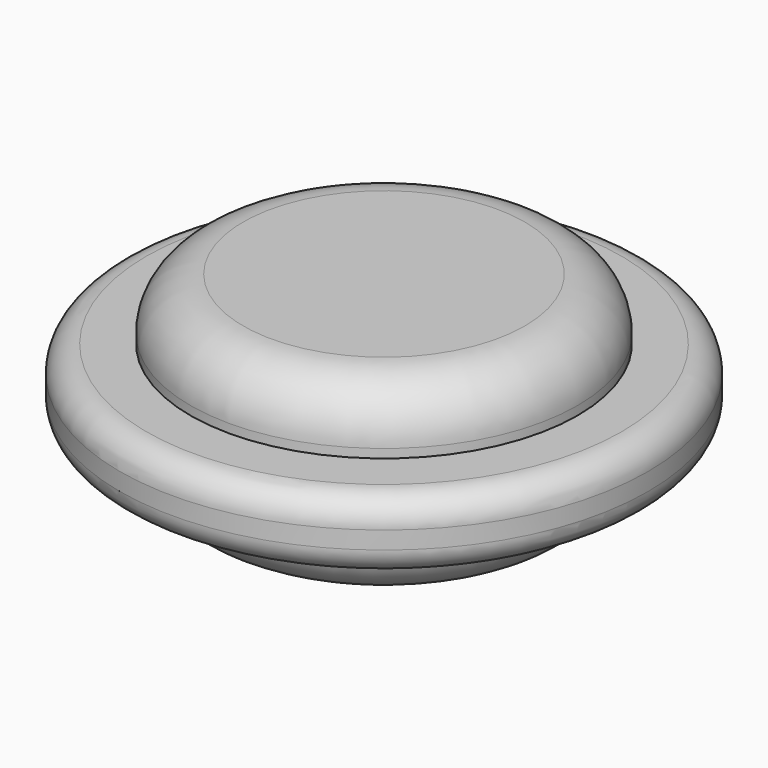
from build123d import *

# Parameters (mm, degrees)
F2_R     = 15
F2_R_2   = 11
F3_DEPTH = 2
F4_R     = 11
F5_DEPTH = 5.5
F6_R     = 3
F7_R     = 1.5
F8_R     = 15
F8_R_2   = 10.75
F9_DEPTH = 2


with BuildPart() as f3:
    # F2 (on Top) → F3 (new body, symmetric)
    with BuildSketch(Plane.XY):
        Circle(F2_R)
        Circle(F2_R_2, mode=Mode.SUBTRACT)
    extrude(amount=F3_DEPTH, both=True)

    # F7
    f7_edges = [f3.edges().sort_by_distance(p)[0] for p in [
        (-15, 0, -2),
        (15, 0, 0),
        (-15, 0, 2),
    ]]
    fillet(f7_edges, radius=F7_R)


with BuildPart() as f5:
    # F4 (on Top) → F5 (new body, symmetric)
    with BuildSketch(Plane.XY):
        Circle(F4_R)
    extrude(amount=F5_DEPTH, both=True)

    # F6
    f6_edges = [f5.edges().sort_by_distance(p)[0] for p in [
        (-11, 0, 5.5),
        (-11, 0, -5.5),
    ]]
    fillet(f6_edges, radius=F6_R)


with BuildPart() as f9:
    # F8 (on Top) → F9 (new body, symmetric)
    with BuildSketch(Plane.XY):
        Circle(F8_R)
        Circle(F8_R_2, mode=Mode.SUBTRACT)
    extrude(amount=F9_DEPTH, both=True)


with BuildPart() as f5_1:
    add(f5.part)

    # F10: cut F9
    add(f9.part, mode=Mode.SUBTRACT)


solid = Compound([f3.part, f5_1.part])
